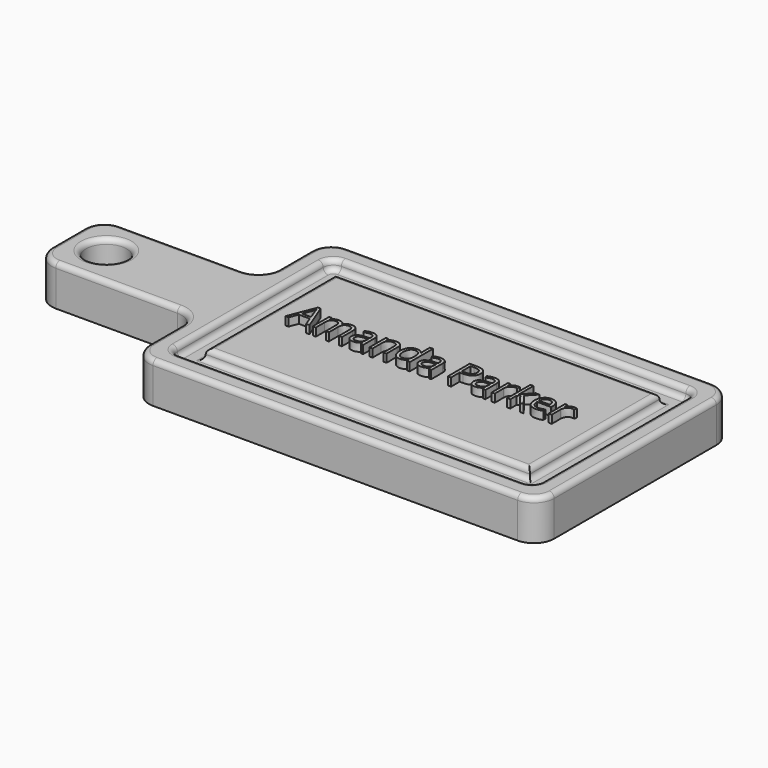
from build123d import *

# Parameters (mm, degrees)
F0_W         = 101.6
F0_H         = 50.8
F1_DEPTH     = 25.4
F2_R         = 12.7
F3_DEPTH     = 25.4
F5_DEPTH     = 6.35
F6_R         = 6.35
F7_R         = 12.7
F8_R         = 3.17499
F9_TEXT_SIZE = 23.926432348
F10_DEPTH    = 5.08


# Not quite as in the source:
# - a fillet or chamfer is up to 0.001 mm smaller than in the source, because OpenCascade refuses the exact size
# - Text() gives the source's letters only with a copy of the font that has no kerning and outlines rounded to 1/6400 em; it was checked with that copy


with BuildPart() as f1:
    # F0 (on Top) → F1 (new body)
    with BuildSketch(Plane.XY):
        Polygon((0, 50.8), (0, 0), (254, 0), (254, 152.4), (0, 152.4), (0, 101.6), align=None)
        with Locations((-50.8, 76.2)):
            Rectangle(F0_W, F0_H)
    extrude(amount=F1_DEPTH)

    # F2 (on face) → F3 (cut)
    with BuildSketch(Plane.XY.offset(25.4)):
        with Locations((-77.5512754917, 76.2)):
            Circle(F2_R)
    extrude(amount=-F3_DEPTH, mode=Mode.SUBTRACT)

    # F4 (on face) → F5 (cut)
    with BuildSketch(Plane.XY.offset(25.4)):
        Polygon((12.7000044823, 50.8), (12.7000044823, 12.7000044823), (241.2999955177, 12.7000044823), (241.2999955177, 139.6999955177), (12.7000044823, 139.6999955177), (12.7000044823, 101.6), align=None)
        Polygon((25.400010848, 50.8), (25.400010848, 101.6), (25.400010848, 126.999989152), (228.599989152, 126.999989152), (228.599989152, 25.400010848), (25.400010848, 25.400010848), align=None, mode=Mode.SUBTRACT)
    extrude(amount=-F5_DEPTH, mode=Mode.SUBTRACT)

    # F6
    f6_edges = [f1.edges().sort_by_distance(p)[0] for p in [
        (12.700004, 139.699996, 22.225),
        (12.700004, 12.700004, 22.225),
        (241.299996, 139.699996, 22.225),
        (241.299996, 12.700004, 22.225),
    ]]
    fillet(f6_edges, radius=F6_R)

    # F7
    f7_edges = [f1.edges().sort_by_distance(p)[0] for p in [
        (0, 0, 12.7),
        (0, 152.4, 12.7),
        (254, 152.4, 12.7),
        (254, 0, 12.7),
        (-101.6, 101.6, 12.7),
        (-101.6, 50.8, 12.7),
        (0, 101.6, 12.7),
        (0, 50.8, 12.7),
    ]]
    fillet(f7_edges, radius=F7_R)

    # F8 (radius 3.175 in the source; OpenCascade refuses exactly that, so slightly less here)
    f8_edges = [f1.edges().sort_by_distance(p)[0] for p in [
        (127, 0, 25.4),
        (127, 12.700004, 25.4),
        (127, 25.400011, 25.4),
        (228.599989, 76.2, 25.4),
        (127, 126.999989, 25.4),
        (25.400011, 76.2, 25.4),
        (12.700004, 76.2, 19.05),
        (127, 25.400011, 19.05),
        (25.400011, 76.2, 19.05),
        (127, 126.999989, 19.05),
        (228.599989, 76.2, 19.05),
        (-64.851275, 76.2, 12.7),
        (-90.251275, 76.2, 25.4),
        (-90.251275, 76.2, 0),
    ]]
    fillet(f8_edges, radius=F8_R)

    # F9 (on face) → F10 (join)
    with BuildSketch(Plane.XY.offset(25.4)):
        with Locations((40.4539033771, 68.9651072025)):
            Text('Amanda Parker', F9_TEXT_SIZE, font='Open Sans', text_align=(TextAlign.LEFT, TextAlign.BOTTOM))
    extrude(amount=F10_DEPTH)


solid = f1.part
